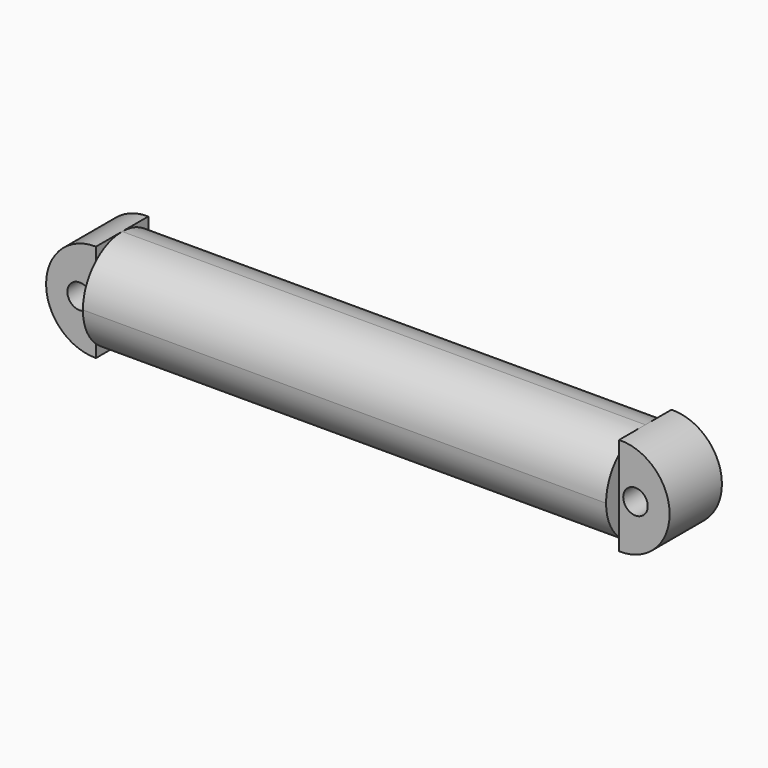
from build123d import *

# Parameters (mm, degrees)
F0_W     = 203.2
F0_H     = 38.1
F1_DEPTH = 19.05
F2_R     = 19.04999
F4_DEPTH = 12.7
F5_R     = 4.7625
F6_DEPTH = 12.7


# Not quite as in the source:
# - a fillet or chamfer is up to 0.001 mm smaller than in the source, because OpenCascade refuses the exact size


with BuildPart() as f1:
    # F0 (on Front) → F1 (new body, symmetric)
    with BuildSketch(Plane.XZ):
        Rectangle(F0_W, F0_H)
    extrude(amount=F1_DEPTH, both=True)

    # F2 (radius 19.05 in the source; OpenCascade refuses exactly that, so slightly less here)
    f2_edges = [f1.edges().sort_by_distance(p)[0] for p in [
        (0, -19.05, 19.05),
        (0, 19.05, 19.05),
        (0, 19.05, -19.05),
        (0, -19.05, -19.05),
    ]]
    fillet(f2_edges, radius=F2_R)

    # F3 (on Front) → F4 (join, symmetric)
    with BuildSketch(Plane.XZ):
        with BuildLine():
            Line((-101.6, -19.0500002354), (-101.6, 0))
            Line((-101.6, 0), (-101.6, 19.05))
            ThreePointArc((-101.6, 19.05), (-120.9801457995, -1.177e-07), (-101.6, -19.0500002354))
        make_face()
        with BuildLine():
            Line((101.6, 19.05), (101.6, 0))
            Line((101.6, 0), (101.6, -19.0500002354))
            ThreePointArc((101.6, -19.0500002354), (121.1996012404, -1.177e-07), (101.6, 19.05))
        make_face()
    extrude(amount=F4_DEPTH, both=True)

    # F5 (on Front) → F6 (cut, symmetric)
    with BuildSketch(Plane.XZ):
        with Locations((-107.95, 0)):
            Circle(F5_R)
        with BuildLine():
            ThreePointArc((112.7125, 0), (107.95, 4.7625), (103.1875, 0))
            ThreePointArc((103.1875, 0), (107.95, -4.7625), (112.7125, 0))
        make_face()
    extrude(amount=F6_DEPTH, both=True, mode=Mode.SUBTRACT)


solid = f1.part
